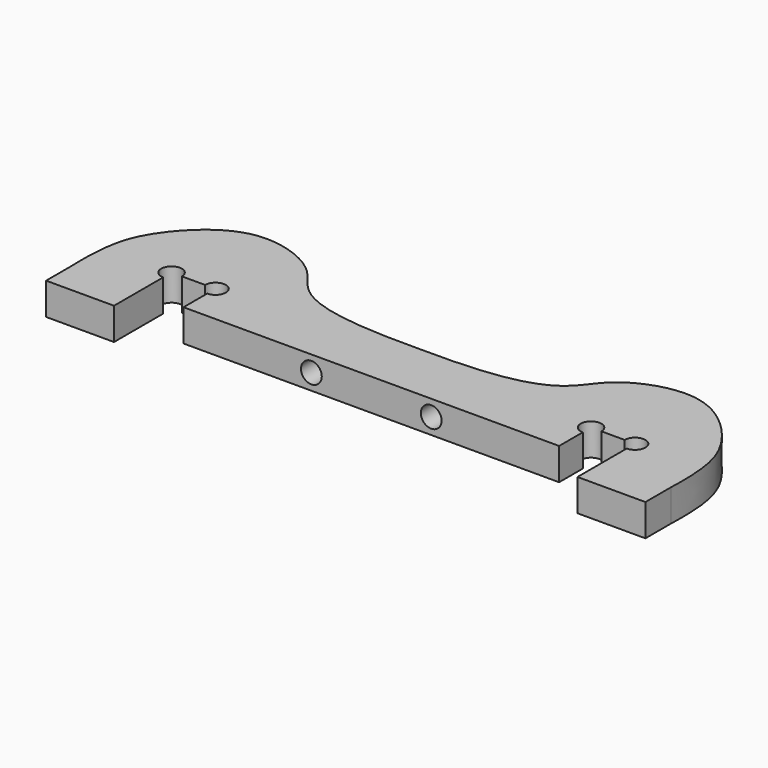
from build123d import *

# Parameters (mm, degrees)
F1_DEPTH  = 8
F2_R      = 2.6
F3_DEPTH  = 32.7754338425
F4_W      = 17
F4_H      = 8
F5_DEPTH  = 8
F6_W      = 11
F6_H      = 8
F7_DEPTH  = 10
F10_DEPTH = 8.0010001


# Not quite as in the source:
# - a feature names something its author has since deleted; it is built from what else it names


with BuildPart() as f1:
    # F0 (on Top) → F1 (new body)
    with BuildSketch(Plane.XY):
        with BuildLine():
            Line((-75, 0), (0, 0))
            Line((0, 0), (0, 15))
            add(Edge.make_bspline(
                [(0, 15), (-33.8492020965, 14.5203908905), (-31.1904909634, 26.878043416), (-56.3916650053, 36.3544882745), (-72.7604456377, 21.0379339388), (-75.3937876263, 11.3815652157), (-75, 0)],
                knots=[0, 0, 0, 0, 0.3227401515, 0.539922816, 0.7595547121, 1, 1, 1, 1], degree=3))
        make_face()
    extrude(amount=F1_DEPTH)

    # F2 (on face) → F3 (cut, through all)
    with BuildSketch(Plane.XZ):
        with Locations((-15, 4)):
            Circle(F2_R)
        with Locations((15, 4)):
            Circle(F2_R)
    extrude(amount=-F3_DEPTH, mode=Mode.SUBTRACT)

    # F4 (on face) → F5 (join)
    with BuildSketch(Plane.XZ):
        with Locations((-66.5, 4)):
            Rectangle(F4_W, F4_H)
    extrude(amount=F5_DEPTH)

    # F6 (on face) → F7 (cut)
    with BuildSketch(Plane.XZ):
        with Locations((-52.5, 4)):
            Rectangle(F6_W, F6_H)
    extrude(amount=-F7_DEPTH, mode=Mode.SUBTRACT)

    # F8: F1 across face


with BuildPart() as f1_1:
    add(f1.part)
    add(f1.part.mirror(Plane(origin=(0, 7.5, 4), x_dir=(0, 1, 0), z_dir=(1, 0, 0))))

    # F9 (on face) → F10 (cut, through all)
    with BuildSketch(Plane.XY.offset(8)):
        with BuildLine():
            ThreePointArc((58, 7.4), (59.8384776311, 8.1615223689), (60.6, 10))
            ThreePointArc((60.6, 10), (58, 12.6), (55.4, 10))
            Line((55.4, 10), (58, 10))
            Line((58, 10), (58, 7.4))
        make_face()
        with BuildLine():
            Line((47, 10), (49.6, 10))
            ThreePointArc((49.6, 10), (45.1615223689, 11.8384776311), (47, 7.4))
            Line((47, 7.4), (47, 10))
        make_face()
        with BuildLine():
            Line((-47, 10), (-47, 7.4))
            ThreePointArc((-47, 7.4), (-45.1615223689, 8.1615223689), (-44.4, 10))
            ThreePointArc((-44.4, 10), (-47, 12.6), (-49.6, 10))
            Line((-49.6, 10), (-47, 10))
        make_face()
        with BuildLine():
            Line((-58, 10), (-55.4, 10))
            ThreePointArc((-55.4, 10), (-59.8384776311, 11.8384776311), (-58, 7.4))
            Line((-58, 7.4), (-58, 10))
        make_face()
    extrude(amount=-F10_DEPTH, mode=Mode.SUBTRACT)


solid = f1_1.part
